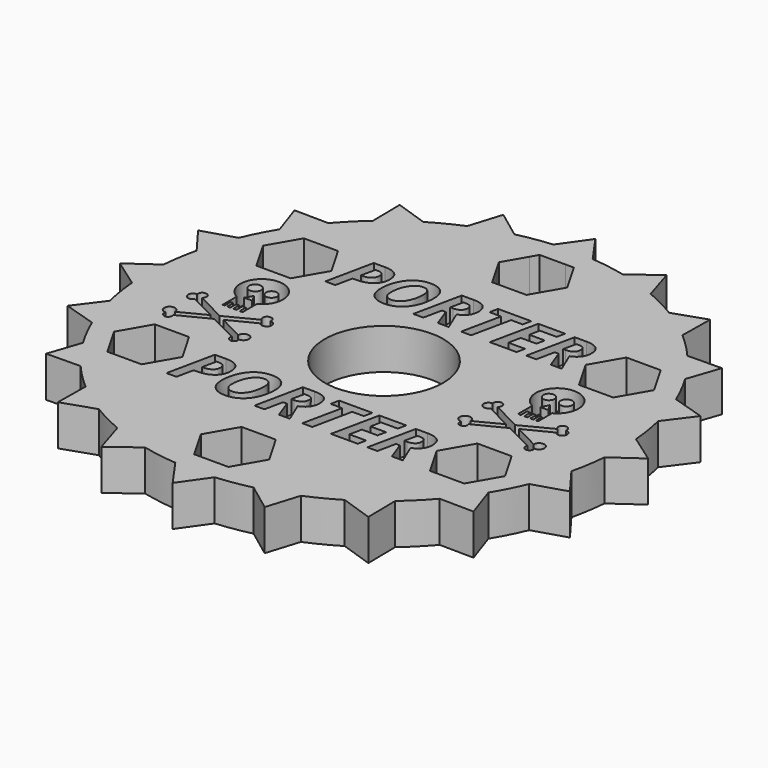
from build123d import *

# Parameters (mm, degrees)
F0_R         = 44.45
F0_R_2       = 11.1125
F1_DEPTH     = 7.62
F3_DEPTH     = 25.4
F4_TEXT_SIZE = 12.5915019049
F5_DEPTH     = 3.81
F7_DEPTH     = 7.62
F8_R         = 1.0488631735
F8_R_2       = 1.1204571862
F9_DEPTH     = 3.81


# Not quite as in the source:
# - Text() gives the source's letters only with a copy of the font that has no kerning and outlines rounded to 1/6400 em; it was checked with that copy


with BuildPart() as f1:
    # F0 (on Top) → F1 (new body)
    with BuildSketch(Plane.XY):
        Circle(F0_R)
        Circle(F0_R_2, mode=Mode.SUBTRACT)
        Polygon((3.2090448956, 40.4805902424), (6.4158047307, 34.9236807198), (3.2067598352, 29.3680904774), (-3.2090448956, 29.3694097576), (-6.4158047307, 34.9263192802), (-3.2067598352, 40.4819095226), align=None, mode=Mode.SUBTRACT)
    extrude(amount=F1_DEPTH)

    # F2 (on face) → F3 (cut)
    with BuildSketch(Plane(origin=(0, 0, 0), x_dir=(1, 0, 0), z_dir=(0, 0, -1))):
        Polygon((0, -29.3694095226), (-3.2063789918, -29.3687501175), (-6.4150430439, -34.9236807198), (-3.2086640522, -40.4799306023), (3.2063789918, -40.4812498825), (6.4150430439, -34.9263192802), (3.2086640522, -29.3700693977), align=None)
        Polygon((27.037273175, -23.0174306023), (33.4523162189, -23.0187498825), (36.6609802711, -17.4638192802), (33.4546012793, -11.9075693977), (27.0395582354, -11.9062501175), (23.8308941832, -17.4611807198), align=None)
        Polygon((33.4523162189, 11.9062501175), (36.6609802711, 17.4611807198), (33.4546012793, 23.0174306023), (27.0395582354, 23.0187498825), (23.8308941832, 17.4638192802), (27.037273175, 11.9075693977), align=None)
        Polygon((6.4150430439, 34.9236807198), (3.2086640522, 40.4799306023), (-3.2063789918, 40.4812498825), (-6.4150430439, 34.9263192802), (-3.2086640522, 29.3700693977), (3.2063789918, 29.3687501175), align=None)
        Polygon((-27.037273175, 23.0174306023), (-33.4523162189, 23.0187498825), (-36.6609802711, 17.4638192802), (-33.4546012793, 11.9075693977), (-27.0395582354, 11.9062501175), (-23.8308941832, 17.4611807198), align=None)
        Polygon((-33.4523162189, -11.9062501175), (-36.6609802711, -17.4611807198), (-33.4546012793, -23.0174306023), (-27.0395582354, -23.0187498825), (-23.8308941832, -17.4638192802), (-27.037273175, -11.9075693977), align=None)
    extrude(amount=-F3_DEPTH, mode=Mode.SUBTRACT)

    # F4 (on face) → F5 (cut)
    with BuildSketch(Plane.XY.offset(7.62)):
        with Locations((-22.7911546826, -22.9155511285)):
            Text('PORTER', F4_TEXT_SIZE, font='Open Sans', font_style=FontStyle.BOLDITALIC, text_align=(TextAlign.LEFT, TextAlign.BOTTOM))
        with Locations((-22.7911546826, 14.3201425672)):
            Text('PORTER', F4_TEXT_SIZE, font='Open Sans', font_style=FontStyle.BOLDITALIC, text_align=(TextAlign.LEFT, TextAlign.BOTTOM))
    extrude(amount=-F5_DEPTH, mode=Mode.SUBTRACT)

    # F6 (on face) → F7 (join)
    with BuildSketch(Plane.XY.offset(7.62)):
        Polygon((4.7097750939, 42.8595580161), (0, 49.53), (-4.7097750939, 42.8595580161), align=None)
        Polygon((-8.765069505, 42.2172624804), (-15.3056117314, 47.1058292521), (-17.7235940917, 39.306461393), align=None)
        Polygon((-21.3819280309, 37.4424471482), (-29.113003546, 40.0706117314), (-29.0025042123, 31.9057744646), align=None)
        Polygon((-31.9057744646, 29.0025042123), (-40.0706117314, 29.113003546), (-37.4424471482, 21.3819280309), align=None)
        Polygon((-39.306461393, 17.7235940917), (-47.1058292521, 15.3056117314), (-42.2172624804, 8.765069505), align=None)
        Polygon((-42.8595580161, 4.7097750939), (-49.53, 0), (-42.8595580161, -4.7097750939), align=None)
        Polygon((-42.2172624804, -8.765069505), (-47.1058292521, -15.3056117314), (-39.306461393, -17.7235940917), align=None)
        Polygon((-37.4424471482, -21.3819280309), (-40.0706117314, -29.113003546), (-31.9057744646, -29.0025042123), align=None)
        Polygon((-29.0025042123, -31.9057744646), (-29.113003546, -40.0706117314), (-21.3819280309, -37.4424471482), align=None)
        Polygon((-17.7235940917, -39.306461393), (-15.3056117314, -47.1058292521), (-8.765069505, -42.2172624804), align=None)
        Polygon((-4.7097750939, -42.8595580161), (0, -49.53), (4.7097750939, -42.8595580161), align=None)
        Polygon((8.765069505, -42.2172624804), (15.3056117314, -47.1058292521), (17.7235940917, -39.306461393), align=None)
        Polygon((21.3819280309, -37.4424471482), (29.113003546, -40.0706117314), (29.0025042123, -31.9057744646), align=None)
        Polygon((31.9057744646, -29.0025042123), (40.0706117314, -29.113003546), (37.4424471482, -21.3819280309), align=None)
        Polygon((39.306461393, -17.7235940917), (47.1058292521, -15.3056117314), (42.2172624804, -8.765069505), align=None)
        Polygon((42.8595580161, -4.7097750939), (49.53, 0), (42.8595580161, 4.7097750939), align=None)
        Polygon((42.2172624804, 8.765069505), (47.1058292521, 15.3056117314), (39.306461393, 17.7235940917), align=None)
        Polygon((37.4424471482, 21.3819280309), (40.0706117314, 29.113003546), (31.9057744646, 29.0025042123), align=None)
        Polygon((29.0025042123, 31.9057744646), (29.113003546, 40.0706117314), (21.3819280309, 37.4424471482), align=None)
        Polygon((17.7235940917, 39.306461393), (15.3056117314, 47.1058292521), (8.765069505, 42.2172624804), align=None)
    extrude(amount=-F7_DEPTH)

    # F8 (on face) → F9 (cut)
    with BuildSketch(Plane.XY.offset(7.62)):
        with BuildLine():
            Line((29.5799607252, -0.8705060268), (29.5799607252, 2.4343234904))
            ThreePointArc((29.5799607252, 2.4343234904), (27.7043441151, 9.9656114537), (25.8287275051, 2.4343234904))
            Line((25.8287275051, 2.4343234904), (25.8287275051, -0.8705060268))
            Line((25.8287275051, -0.8705060268), (26.3680713092, -0.8705060268))
            Line((26.3680713092, -0.8705060268), (26.3680713092, 0.5669021826))
            Line((26.3680713092, 0.5669021826), (26.9731087451, 0.5669021826))
            Line((26.9731087451, 0.5669021826), (26.9731087451, -0.8705060268))
            Line((26.9731087451, -0.8705060268), (27.578146181, -0.8705060268))
            Line((27.578146181, -0.8705060268), (27.578146181, 0.5063986369))
            Line((27.578146181, 0.5063986369), (28.1226793145, 0.5063986369))
            Line((28.1226793145, 0.5063986369), (28.1226793145, -0.8705060268))
            Line((28.1226793145, -0.8705060268), (28.6974655305, -0.8705060268))
            Line((28.6974655305, -0.8705060268), (28.6974655305, 0.5366501478))
            Line((28.6974655305, 0.5366501478), (29.1814943616, 0.5366501478))
            Line((29.1814943616, 0.5366501478), (29.1814943616, -0.8705060268))
            Line((29.1814943616, -0.8705060268), (29.5799607252, -0.8705060268))
        make_face()
        Polygon((27.0138112669, 2.8681189483), (27.7260942225, 4.2418076387), (28.5146934752, 2.8681189483), align=None, mode=Mode.SUBTRACT)
        with Locations((26.0056936954, 6.1529453574)):
            Circle(F8_R, mode=Mode.SUBTRACT)
        with Locations((29.1855269884, 6.2801384097)):
            Circle(F8_R_2, mode=Mode.SUBTRACT)
        with BuildLine():
            Line((27.7043441151, -3.8872638683), (22.1235017233, -0.9998340945))
            ThreePointArc((22.1235017233, -0.9998340945), (21.8770357577, 0.4075525472), (20.836552531, -0.57167025))
            ThreePointArc((20.836552531, -0.57167025), (19.9641021542, -1.8864805545), (21.5386526765, -1.9898558395))
            Line((21.5386526765, -1.9898558395), (26.5047850896, -4.5078946266))
            Line((26.5047850896, -4.5078946266), (21.7755964512, -6.9546937157))
            ThreePointArc((21.7755964512, -6.9546937157), (20.0323957938, -6.2611076708), (20.8363966361, -7.9562161568))
            ThreePointArc((20.8363966361, -7.9562161568), (21.5520995831, -8.9975635998), (22.1948457475, -7.9096699591))
            Line((22.1948457475, -7.9096699591), (27.7043441151, -5.116121694))
            Line((27.7043441151, -5.116121694), (33.2138424828, -7.9096699591))
            ThreePointArc((33.2138424828, -7.9096699591), (33.8565886472, -8.9975635998), (34.5722915942, -7.9562161568))
            ThreePointArc((34.5722915942, -7.9562161568), (35.3762924365, -6.2611076708), (33.6330917791, -6.9546937157))
            Line((33.6330917791, -6.9546937157), (28.9039031407, -4.5078946266))
            Line((28.9039031407, -4.5078946266), (33.8700355538, -1.9898558395))
            ThreePointArc((33.8700355538, -1.9898558395), (35.4445860761, -1.8864805545), (34.5721356992, -0.57167025))
            ThreePointArc((34.5721356992, -0.57167025), (33.5316524726, 0.4075525472), (33.285186507, -0.9998340945))
            Line((33.285186507, -0.9998340945), (27.7043441151, -3.8872638683))
        make_face()
        with BuildLine():
            Line((-29.1814943616, 0.5366501478), (-28.6974655305, 0.5366501478))
            Line((-28.6974655305, 0.5366501478), (-28.6974655305, -0.8705060268))
            Line((-28.6974655305, -0.8705060268), (-28.1226793145, -0.8705060268))
            Line((-28.1226793145, -0.8705060268), (-28.1226793145, 0.5063986369))
            Line((-28.1226793145, 0.5063986369), (-27.578146181, 0.5063986369))
            Line((-27.578146181, 0.5063986369), (-27.578146181, -0.8705060268))
            Line((-27.578146181, -0.8705060268), (-26.9731087451, -0.8705060268))
            Line((-26.9731087451, -0.8705060268), (-26.9731087451, 0.5669021826))
            Line((-26.9731087451, 0.5669021826), (-26.3680713092, 0.5669021826))
            Line((-26.3680713092, 0.5669021826), (-26.3680713092, -0.8705060268))
            Line((-26.3680713092, -0.8705060268), (-25.8287275051, -0.8705060268))
            Line((-25.8287275051, -0.8705060268), (-25.8287275051, 2.4343234904))
            ThreePointArc((-25.8287275051, 2.4343234904), (-27.7043441151, 9.9656114537), (-29.5799607252, 2.4343234904))
            Line((-29.5799607252, 2.4343234904), (-29.5799607252, -0.8705060268))
            Line((-29.5799607252, -0.8705060268), (-29.1814943616, -0.8705060268))
            Line((-29.1814943616, -0.8705060268), (-29.1814943616, 0.5366501478))
        make_face()
        Polygon((-27.0138112669, 2.8681189483), (-28.5146934752, 2.8681189483), (-27.7260942225, 4.2418076387), align=None, mode=Mode.SUBTRACT)
        with Locations((-29.1855269884, 6.2801384097)):
            Circle(F8_R_2, mode=Mode.SUBTRACT)
        with Locations((-26.0056936954, 6.1529453574)):
            Circle(F8_R, mode=Mode.SUBTRACT)
        with BuildLine():
            ThreePointArc((-20.836552531, -0.57167025), (-21.8770357577, 0.4075525472), (-22.1235017233, -0.9998340945))
            Line((-22.1235017233, -0.9998340945), (-27.7043441151, -3.8872638683))
            Line((-27.7043441151, -3.8872638683), (-33.285186507, -0.9998340945))
            ThreePointArc((-33.285186507, -0.9998340945), (-33.5316524726, 0.4075525472), (-34.5721356992, -0.57167025))
            ThreePointArc((-34.5721356992, -0.57167025), (-35.4445860761, -1.8864805545), (-33.8700355538, -1.9898558395))
            Line((-33.8700355538, -1.9898558395), (-28.9039031407, -4.5078946266))
            Line((-28.9039031407, -4.5078946266), (-33.6330917791, -6.9546937157))
            ThreePointArc((-33.6330917791, -6.9546937157), (-35.3762924365, -6.2611076708), (-34.5722915942, -7.9562161568))
            ThreePointArc((-34.5722915942, -7.9562161568), (-33.8565886472, -8.9975635998), (-33.2138424828, -7.9096699591))
            Line((-33.2138424828, -7.9096699591), (-27.7043441151, -5.116121694))
            Line((-27.7043441151, -5.116121694), (-22.1948457475, -7.9096699591))
            ThreePointArc((-22.1948457475, -7.9096699591), (-21.5520995831, -8.9975635998), (-20.8363966361, -7.9562161568))
            ThreePointArc((-20.8363966361, -7.9562161568), (-20.0323957938, -6.2611076708), (-21.7755964512, -6.9546937157))
            Line((-21.7755964512, -6.9546937157), (-26.5047850896, -4.5078946266))
            Line((-26.5047850896, -4.5078946266), (-21.5386526765, -1.9898558395))
            ThreePointArc((-21.5386526765, -1.9898558395), (-19.9641021542, -1.8864805545), (-20.836552531, -0.57167025))
        make_face()
    extrude(amount=-F9_DEPTH, mode=Mode.SUBTRACT)


solid = f1.part
